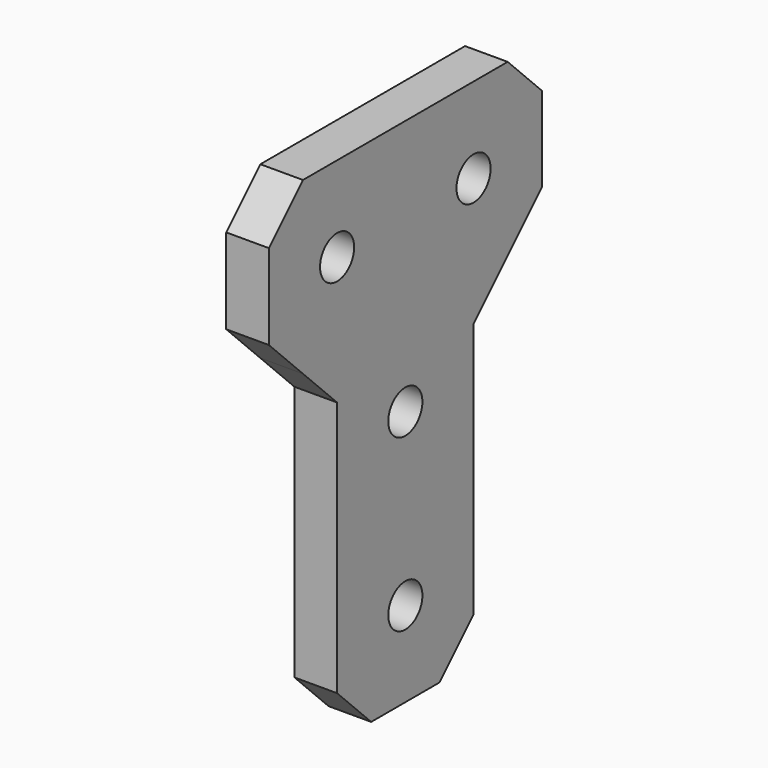
from build123d import *

# Parameters (mm, degrees)
F0_R     = 2.5
F1_DEPTH = 5
F2_SIZE  = 4.99999


# Not quite as in the source:
# - a fillet or chamfer is up to 0.001 mm smaller than in the source, because OpenCascade refuses the exact size


with BuildPart() as f1:
    # F0 (on Right) → F1 (new body)
    with BuildSketch(Plane.YZ):
        Polygon((-10, 0), (10, 0), (10, 40), (20, 40), (20, 60), (-20, 60), (-20, 40), (-10, 40), align=None)
        with Locations((0, 10)):
            Circle(F0_R, mode=Mode.SUBTRACT)
        with Locations((-10, 50)):
            Circle(F0_R, mode=Mode.SUBTRACT)
        with Locations((0, 30)):
            Circle(F0_R, mode=Mode.SUBTRACT)
        with Locations((10, 50)):
            Circle(F0_R, mode=Mode.SUBTRACT)
    extrude(amount=F1_DEPTH)

    # F2 (size 5 in the source; OpenCascade refuses exactly that, so slightly less here)
    f2_edges = [f1.edges().sort_by_distance(p)[0] for p in [
        (2.5, 10, 40),
        (2.5, 20, 40),
        (2.5, 20, 60),
        (2.5, 10, 0),
        (2.5, -10, 0),
        (2.5, -10, 40),
        (2.5, -20, 40),
        (2.5, -20, 60),
    ]]
    chamfer(f2_edges, length=F2_SIZE)


solid = f1.part
